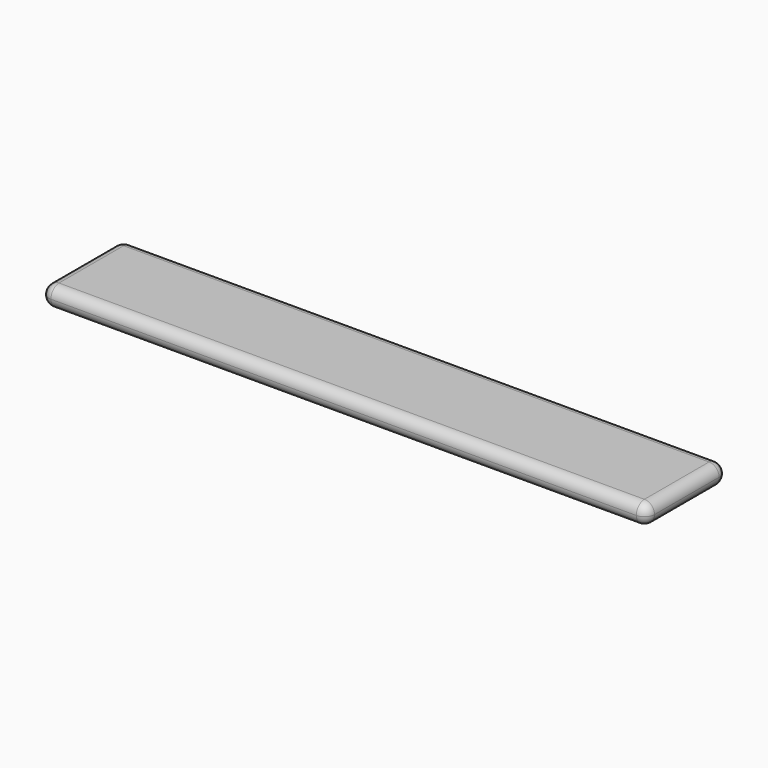
from build123d import *

# Parameters (mm, degrees)
F0_W     = 30
F0_H     = 5
F1_DEPTH = 1
F2_R     = 0.49999


# Not quite as in the source:
# - a fillet or chamfer is up to 0.001 mm smaller than in the source, because OpenCascade refuses the exact size


with BuildPart() as f1:
    # F0 (on Top) → F1 (new body)
    with BuildSketch(Plane.XY):
        with Locations((-35.3688234463, 21.3975507232)):
            Rectangle(F0_W, F0_H)
    extrude(amount=F1_DEPTH)

    # F2 (radius 0.5 in the source; OpenCascade refuses exactly that, so slightly less here)
    f2_edges = [f1.edges().sort_by_distance(p)[0] for p in [
        (-35.368823, 23.897551, 1),
        (-50.368823, 21.397551, 1),
        (-35.368823, 18.897551, 1),
        (-20.368823, 21.397551, 1),
        (-50.368823, 18.897551, 0.5),
        (-20.368823, 18.897551, 0.5),
        (-35.368823, 18.897551, 0),
        (-35.368823, 23.897551, 0),
        (-50.368823, 21.397551, 0),
        (-20.368823, 21.397551, 0),
        (-20.368823, 23.897551, 0.5),
        (-50.368823, 23.897551, 0.5),
    ]]
    fillet(f2_edges, radius=F2_R)


solid = f1.part
